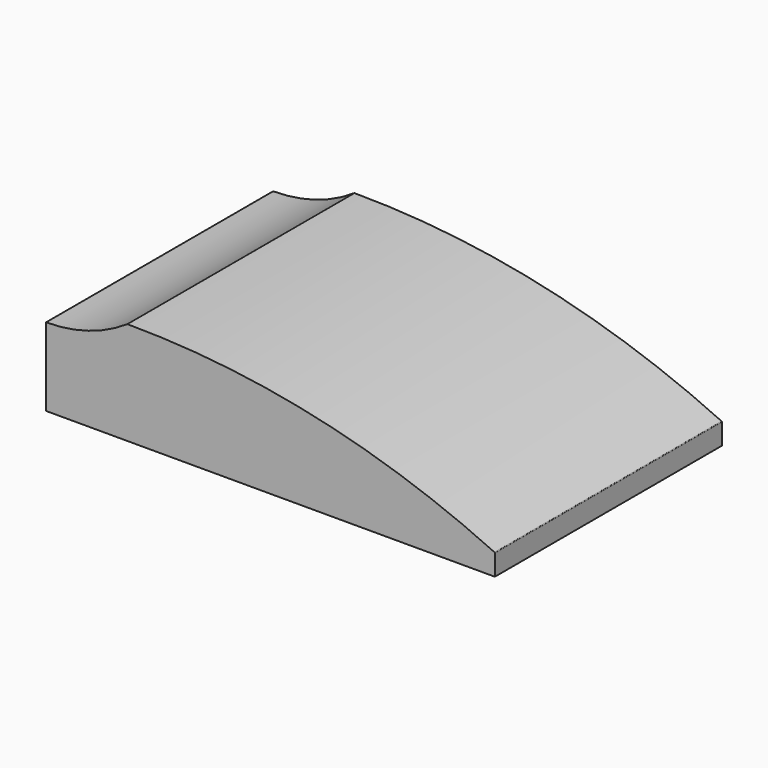
from build123d import *

# Parameters (mm, degrees)
F1_DEPTH = 80


# Not quite as in the source:
# - ends of sketch curves that miss each other by under 0.0002 mm in the source are joined


with BuildPart() as f1:
    # F0 (on Front) → F1 (new body)
    with BuildSketch(Plane.XZ):
        with BuildLine():
            Line((0, 20), (0, 0))
            Line((0, 0), (126.5, 0))
            Line((126.5, 0), (126.5, 5.872634))
            ThreePointArc((126.5, 5.872634), (126.4686827703, 5.9800868873), (126.3845387701, 6.0538885071))
            ThreePointArc((126.3845387701, 6.0538885071), (75.9297421053, 23.1880267358), (22.962901, 28.9999923785))
            ThreePointArc((22.962901, 28.9999923785), (22.9045566452, 28.9913078859), (22.8512831377, 28.9659817952))
            ThreePointArc((22.8512831377, 28.9659817952), (11.9447272771, 23.7801763601), (0, 22))
            Line((0, 22), (0, 20))
        make_face()
    extrude(amount=F1_DEPTH)


solid = f1.part
